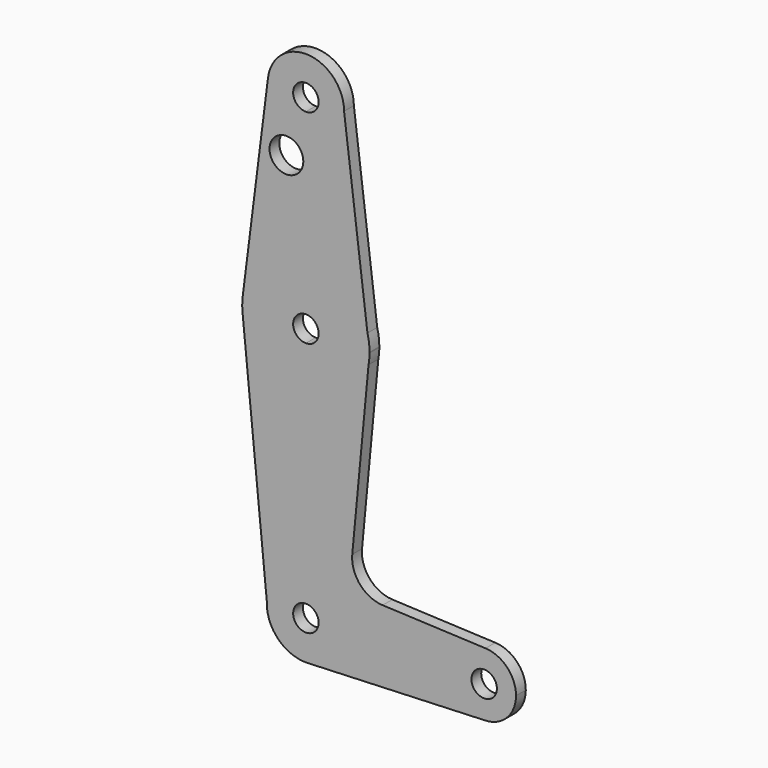
from build123d import *

# Parameters (mm, degrees)
F0_R     = 1.6581186228
F1_DEPTH = 1.2


with BuildPart() as f1:
    # F0 (on Front) → F1 (new body)
    with BuildSketch(Plane.XZ):
        with BuildLine():
            ThreePointArc((1.25, 0), (-0.8838834765, -0.8838834765), (0, 1.25))
            Line((0, 1.25), (0, 3.8304899347))
            ThreePointArc((0, 3.8304899347), (-2.6634496965, 2.7529418545), (-3.8283991196, 0.126543752))
            Line((-3.8283991196, 0.126543752), (-3.7301566118, -0.8709677329))
            ThreePointArc((-3.7301566118, -0.8709677329), (-2.3198010798, -3.048143056), (0.1544652488, -3.8273742471))
            ThreePointArc((0.1544652488, -3.8273742471), (2.7626373921, -2.6533917501), (3.8304899347, 0))
            Line((3.8304899347, 0), (1.25, 0))
        make_face()
        with BuildLine():
            Line((0, 3.8304899347), (0, 1.25))
            ThreePointArc((0, 1.25), (0.8838834765, 0.8838834765), (1.25, 0))
            Line((1.25, 0), (3.8304899347, 0))
            ThreePointArc((3.8304899347, 0), (2.7085654081, 2.7085654081), (0, 3.8304899347))
        make_face()
        with BuildLine():
            ThreePointArc((-3.8283991196, 0.126543752), (-2.6634496965, 2.7529418545), (0, 3.8304899347))
            Line((0, 3.8304899347), (0, 18.75))
            ThreePointArc((0, 18.75), (-4.1368389571, 20.315017242), (-6.2019261398, 24.2262996982))
            Line((-6.2019261398, 24.2262996982), (-3.8283991196, 0.126543752))
        make_face()
        with BuildLine():
            Line((0, 18.75), (0, 3.8304899347))
            ThreePointArc((0, 3.8304899347), (2.7085654081, 2.7085654081), (3.8304899347, 0))
            Line((3.8304899347, 0), (14.375, 0))
            ThreePointArc((14.375, 0), (15.3390218203, 2.257387496), (17.6363109165, 3.122025678))
            Line((17.6363109165, 3.122025678), (7.5319273502, 3.5631936653))
            ThreePointArc((7.5319273502, 3.5631936653), (5.3080013875, 4.6346970575), (4.5523493544, 6.9847941218))
            Line((4.5523493544, 6.9847941218), (6.150289486, 23.8880471063))
            ThreePointArc((6.150289486, 23.8880471063), (4.0070434496, 20.2035322587), (0, 18.75))
        make_face()
        with BuildLine():
            Line((14.375, 0), (3.8304899347, 0))
            ThreePointArc((3.8304899347, 0), (2.7626373921, -2.6533917501), (0.1544652488, -3.8273742471))
            Line((0.1544652488, -3.8273742471), (17.5906089776, -3.1236861259))
            ThreePointArc((17.5906089776, -3.1236861259), (15.3225620623, -2.2415148957), (14.375, 0))
        make_face()
        with BuildLine():
            ThreePointArc((-6.2019261398, 24.2262996982), (-4.1368389571, 20.315017242), (0, 18.75))
            Line((0, 18.75), (0, 23.75))
            ThreePointArc((0, 23.75), (-1.25, 25), (0, 26.25))
            Line((0, 26.25), (0, 31.25))
            ThreePointArc((0, 31.25), (-4.1339767257, 29.6875085527), (-6.2009764026, 25.7812756582))
            ThreePointArc((-6.2009764026, 25.7812756582), (-6.2477972764, 25.1659192352), (-6.2337027111, 24.5489451152))
            Line((-6.2337027111, 24.5489451152), (-6.2019261398, 24.2262996982))
        make_face()
        with BuildLine():
            Line((0, 23.75), (0, 18.75))
            ThreePointArc((0, 18.75), (4.0070434496, 20.2035322587), (6.150289486, 23.8880471063))
            Line((6.150289486, 23.8880471063), (6.2497093523, 24.9397255246))
            Line((6.2497093523, 24.9397255246), (6.0440984205, 26.5910293157))
            ThreePointArc((6.0440984205, 26.5910293157), (3.8156629029, 29.9500723845), (0, 31.25))
            Line((0, 31.25), (0, 26.25))
            ThreePointArc((0, 26.25), (0.8838834765, 25.8838834765), (1.25, 25))
            ThreePointArc((1.25, 25), (0.8838834765, 24.1161165235), (0, 23.75))
        make_face()
        with BuildLine():
            Line((-3.7301566118, -0.8709677329), (-3.8283991196, 0.126543752))
            ThreePointArc((-3.8283991196, 0.126543752), (-3.8120464946, -0.375439294), (-3.7301566118, -0.8709677329))
        make_face()
        with BuildLine():
            ThreePointArc((17.6363109165, 3.122025678), (15.3390218203, 2.257387496), (14.375, 0))
            ThreePointArc((14.375, 0), (15.3225620623, -2.2415148957), (17.5906089776, -3.1236861259))
            ThreePointArc((17.5906089776, -3.1236861259), (19.7415148957, -2.1774379377), (20.625, 0))
            ThreePointArc((20.625, 0), (19.757387496, 2.1609781797), (17.6363109165, 3.122025678))
        make_face()
        with BuildLine():
            ThreePointArc((18.75, 0), (17.5, -1.25), (16.25, 0))
            ThreePointArc((16.25, 0), (17.5, 1.25), (18.75, 0))
        make_face(mode=Mode.SUBTRACT)
        with BuildLine():
            ThreePointArc((-6.2337027111, 24.5489451152), (-6.2199068518, 24.3874163287), (-6.2019261398, 24.2262996982))
            Line((-6.2019261398, 24.2262996982), (-6.2337027111, 24.5489451152))
        make_face()
        with BuildLine():
            Line((6.2497093523, 24.9397255246), (6.150289486, 23.8880471063))
            ThreePointArc((6.150289486, 23.8880471063), (6.222258406, 24.4117820738), (6.2497093523, 24.9397255246))
        make_face()
        with BuildLine():
            Line((6.0440984205, 26.5910293157), (6.2497093523, 24.9397255246))
            ThreePointArc((6.2497093523, 24.9397255246), (6.2499273376, 24.9698624119), (6.25, 25))
            ThreePointArc((6.25, 25), (6.1983108638, 25.8021486371), (6.0440984205, 26.5910293157))
        make_face()
        with BuildLine():
            ThreePointArc((-6.2009764026, 25.7812756582), (-4.1339767257, 29.6875085527), (0, 31.25))
            Line((0, 31.25), (0, 39.38))
            Line((0, 39.38), (0, 41.25))
            ThreePointArc((0, 41.25), (-2.8042828873, 42.5103218104), (-3.7236063691, 45.4441346731))
            Line((-3.7236063691, 45.4441346731), (-6.2009764026, 25.7812756582))
        make_face()
        with Locations((-1.9114875467, 39.38)):
            Circle(F0_R, mode=Mode.SUBTRACT)
        with BuildLine():
            Line((0, 39.38), (0, 31.25))
            ThreePointArc((0, 31.25), (3.8156629029, 29.9500723845), (6.0440984205, 26.5910293157))
            Line((6.0440984205, 26.5910293157), (3.7499672612, 45.015669719))
            ThreePointArc((3.7499672612, 45.015669719), (3.7499918153, 45.0078348766), (3.75, 45))
            ThreePointArc((3.75, 45), (2.6516504294, 42.3483495706), (0, 41.25))
            Line((0, 41.25), (0, 39.38))
        make_face()
        with BuildLine():
            ThreePointArc((3.7499672612, 45.015669719), (0.2146375512, 48.7438523905), (-3.7236063691, 45.4441346731))
            ThreePointArc((-3.7236063691, 45.4441346731), (-2.8042828873, 42.5103218104), (0, 41.25))
            ThreePointArc((0, 41.25), (2.6516504294, 42.3483495706), (3.75, 45))
            ThreePointArc((3.75, 45), (3.7499918153, 45.0078348766), (3.7499672612, 45.015669719))
        make_face()
        with BuildLine():
            ThreePointArc((1.25, 45), (0.8838834765, 44.1161165235), (0, 43.75))
            ThreePointArc((0, 43.75), (-0.8838834765, 45.8838834765), (1.25, 45))
        make_face(mode=Mode.SUBTRACT)
    extrude(amount=F1_DEPTH)


solid = f1.part
